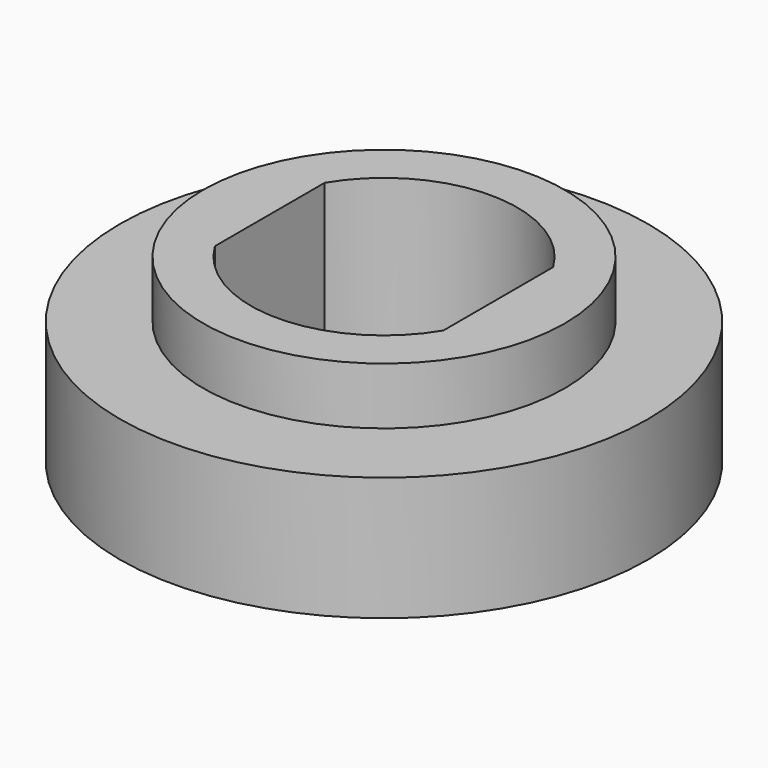
from build123d import *

# Parameters (mm, degrees)
F3_DEPTH = 25
F5_DEPTH = 2


with BuildPart() as f1:
    # F0 (on Front) → F1 (revolve)
    with BuildSketch(Plane.XZ):
        Polygon((19, 0), (0, 0), (0, -17), (16.5, -17), (16.5, -19), (27.75, -19), (27.75, -6), (19, -6), align=None)
    revolve(axis=Axis((0, 0, 0.8052456426), (0, 0, -1)))

    # F2 (on face) → F3 (cut)
    with BuildSketch(Plane.XY):
        with BuildLine():
            Line((-12, 7.2111025509), (-12, -7.2111025509))
            ThreePointArc((-12, -7.2111025509), (0, -14), (12, -7.2111025509))
            Line((12, -7.2111025509), (12, 7.2111025509))
            ThreePointArc((12, 7.2111025509), (0, 14), (-12, 7.2111025509))
        make_face()
    extrude(amount=-F3_DEPTH, mode=Mode.SUBTRACT)

    # F4 (on face) → F5 (cut, through all)
    with BuildSketch(Plane(origin=(0, 0, -19), x_dir=(1, 0, 0), z_dir=(0, 0, -1))):
        with BuildLine():
            Line((-13.1244047484, 10), (-16.1554944214, 10))
            ThreePointArc((-16.1554944214, 10), (-19, 0), (-16.1554944214, -10))
            Line((-16.1554944214, -10), (-13.1244047484, -10))
            ThreePointArc((-13.1244047484, -10), (-16.5, 0), (-13.1244047484, 10))
        make_face()
    extrude(amount=-F5_DEPTH, mode=Mode.SUBTRACT)


solid = f1.part
